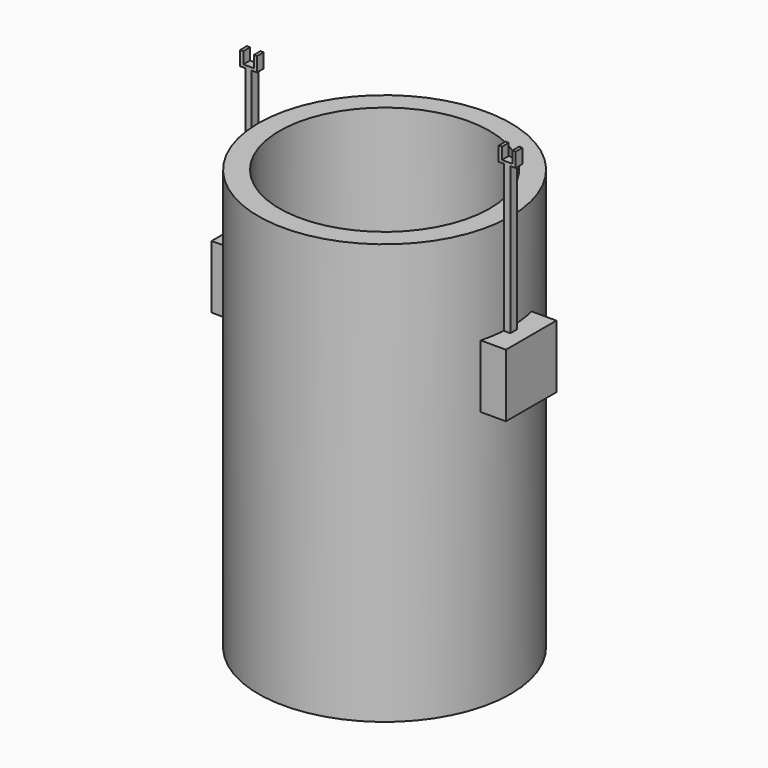
from build123d import *

# Parameters (mm, degrees)
F0_W     = 15.24
F0_H     = 50.8
F2_W     = 7.62
F2_H     = 7.62
F3_DEPTH = 17.78
F5_W     = 0.762
F5_H     = 17.78
F6_DEPTH = 1.016
F8_R     = 12.7
F9_DEPTH = 51.562


# Not quite as in the source:
# - a feature names something its author has since deleted; it is built from what else it names


with BuildPart() as f1:
    # F0 (on Front) → F1 (revolve)
    with BuildSketch(Plane.XZ):
        with Locations((-7.62, 12.8494124473)):
            Rectangle(F0_W, F0_H)
    revolve(axis=Axis((0, 0, 12.8494124473), (0, 0, -1)))

    # F2 (on Right) → F3 (join)
    with BuildSketch(Plane.YZ):
        with Locations((-0.0885345507, 22.6649723111)):
            Rectangle(F2_W, F2_H)
    extrude(amount=F3_DEPTH)

    # F4: F1 across plane


with BuildPart() as f1_1:
    add(f1.part)
    add(f1.part.mirror(Plane.YZ))

    # F5 (on Front) → F6 (join)
    with BuildSketch(Plane.XZ):
        Polygon((15.2397256883, 44.2549723111), (16.0017256883, 44.2549723111), (16.6367256883, 44.2549723111), (16.6367256883, 45.9895022213), (16.2511286259, 45.9895022213), (16.2511286259, 44.5822738111), (14.9926585078, 44.5822738111), (14.9926585078, 45.9895022213), (14.6047256883, 45.9895022213), (14.6047256883, 44.2549723111), align=None)
        with Locations((15.6207256883, 35.3649723111)):
            Rectangle(F5_W, F5_H)
    extrude(amount=F6_DEPTH)

    # F7: F1 across plane


with BuildPart() as f1_2:
    add(f1_1.part)
    add(f1_1.part.mirror(Plane.YZ))

    # F8 (on Top) → F9 (cut)
    with BuildSketch(Plane.XY):
        Circle(F8_R)
    extrude(amount=F9_DEPTH, mode=Mode.SUBTRACT)


solid = f1_2.part
